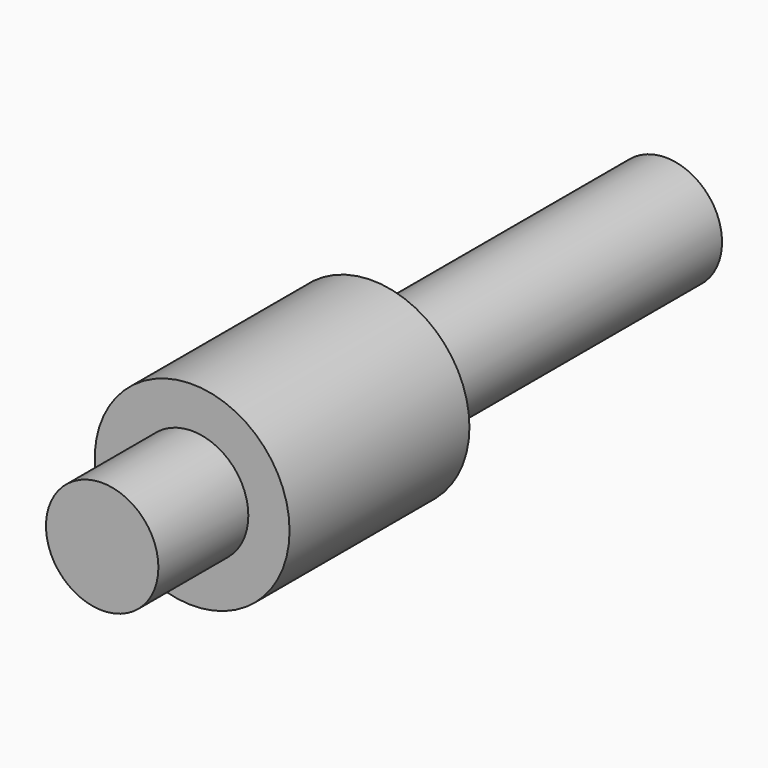
from build123d import *

# Parameters (mm, degrees)
F0_R     = 13
F1_DEPTH = 94
F2_R     = 13
F2_R_2   = 7.5
F3_DEPTH = 15
F4_R     = 13
F4_R_2   = 7.5
F5_DEPTH = 49


with BuildPart() as f1:
    # F0 (on Front) → F1 (new body)
    with BuildSketch(Plane.XZ):
        Circle(F0_R)
    extrude(amount=F1_DEPTH)

    # F2 (on face) → F3 (cut)
    with BuildSketch(Plane.XZ.offset(94)):
        Circle(F2_R)
        Circle(F2_R_2, mode=Mode.SUBTRACT)
    extrude(amount=-F3_DEPTH, mode=Mode.SUBTRACT)

    # F4 (on face) → F5 (cut)
    with BuildSketch(Plane(origin=(0, 0, 0), x_dir=(-1, 0, 0), z_dir=(0, 1, 0))):
        Circle(F4_R)
        Circle(F4_R_2, mode=Mode.SUBTRACT)
    extrude(amount=-F5_DEPTH, mode=Mode.SUBTRACT)


solid = f1.part
